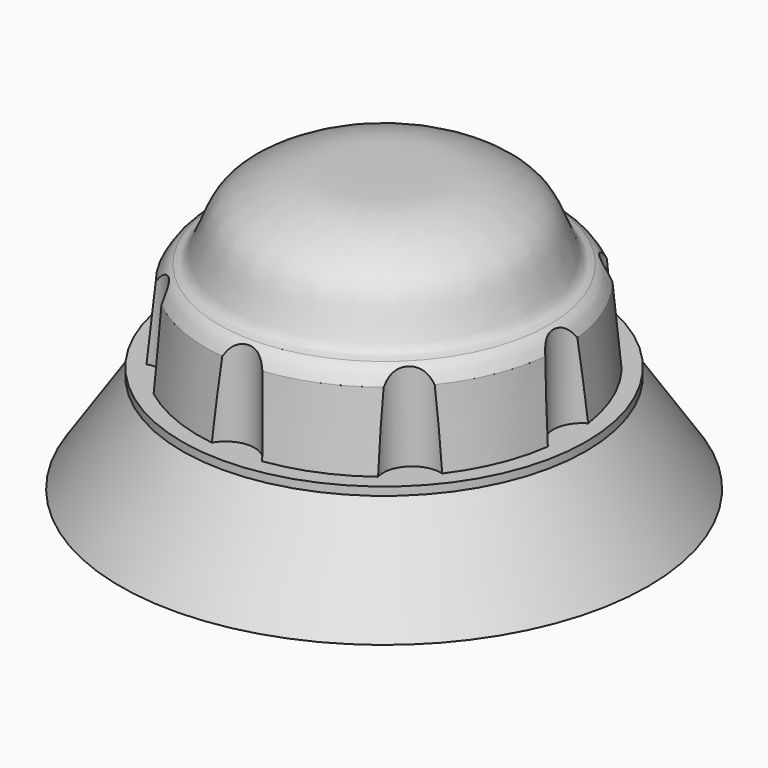
from build123d import *

# Parameters (mm, degrees)
F2_R     = 44.45
F3_DEPTH = 152.4


with BuildPart() as f1:
    # F0 (on Front) → F1 (revolve)
    with BuildSketch(Plane.XZ):
        Polygon((0, 152.4), (0, 0), (406.4, 0), (304.8, 152.4), align=None)
        with BuildLine():
            Line((0, 304.8), (0, 152.4))
            Line((0, 152.4), (304.8, 152.4))
            Line((304.8, 152.4), (311.15, 152.4))
            Line((311.15, 152.4), (311.15, 165.1))
            Line((311.15, 165.1), (285.75, 165.1))
            Line((285.75, 165.1), (274.5597064495, 280.7071506977))
            add(Edge.make_bspline(
                [(274.5597064495, 280.7071506977), (271.7412931371, 285.8037865906), (266.3064654877, 295.6317765268), (258.3550352472, 302.9362996616), (254, 304.8)],
                knots=[0, 0, 0, 0, 0.0771596923, 0.1487892593, 0.1487892593, 0.1487892593, 0.1487892593], degree=3))
            Line((254, 304.8), (0, 304.8))
        make_face()
        with BuildLine():
            Line((0, 432.1574568748), (0, 304.8))
            Line((0, 304.8), (254, 304.8))
            add(Edge.make_bspline(
                [(254, 304.8), (249.5133226892, 306.7200354412), (234.5546852881, 307.2114964849), (217.4700462275, 371.4836376253), (189.2452236448, 397.5288625798), (151.6517387873, 417.6984471616), (107.5702368284, 431.0904789048), (68.3418151338, 432.3167053391), (24.8362806494, 432.2153297824), (0, 432.1574568748)],
                knots=[0.1487892593, 0.1487892593, 0.1487892593, 0.1487892593, 0.222584013, 0.3675456115, 0.4848887913, 0.6047642941, 0.729359126, 0.8454975262, 1, 1, 1, 1], degree=3))
        make_face()
    revolve(axis=Axis((0, 0, 228.6), (0, 0, 1)))

    # F2 (on face) → F3 (cut)
    with BuildSketch(Plane.XY.offset(165.1)):
        with Locations((0, 304.8)):
            Circle(F2_R)
        with Locations((-215.5261469057, 215.5261469057)):
            Circle(F2_R)
        with Locations((-304.8, 0)):
            Circle(F2_R)
        with Locations((-215.5261469057, -215.5261469057)):
            Circle(F2_R)
        with Locations((0, -304.8)):
            Circle(F2_R)
        with Locations((215.5261469057, -215.5261469057)):
            Circle(F2_R)
        with Locations((304.8, 0)):
            Circle(F2_R)
        with Locations((215.5261469057, 215.5261469057)):
            Circle(F2_R)
    extrude(amount=F3_DEPTH, mode=Mode.SUBTRACT)


solid = f1.part
